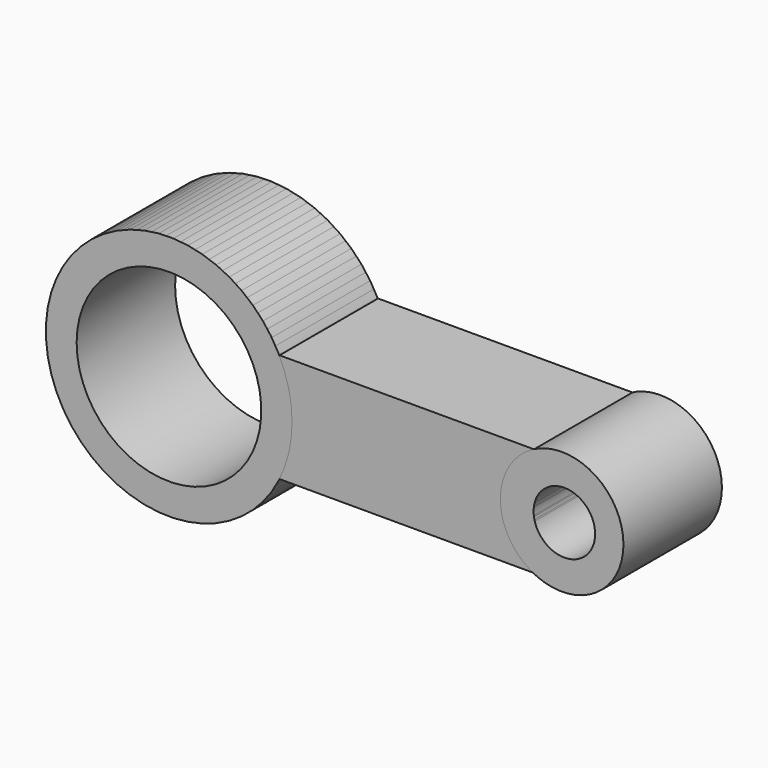
from build123d import *

# Parameters (mm, degrees)
F3_DEPTH   = 12.7
F0_R       = 12.7
F0_R_2     = 6.35
F5_D       = 19.05
F5_DEPTH   = 25.4
F5_TIP     = 5.7231973962
F5_2_D     = 19.05
F5_2_DEPTH = 25.4
F5_2_TIP   = 5.7231973962
F7_D       = 6.35
F7_DEPTH   = 12.7
F7_TIP     = 1.9077324654
F7_2_D     = 6.35
F7_2_DEPTH = 12.7
F7_2_TIP   = 1.9077324654


with BuildPart() as f3:
    # F1 (on face) → F3 (new body)
    with BuildSketch(Plane.XZ):
        with BuildLine():
            Line((37.7772264183, 5.648068618), (11.4167341962, 5.648068618))
            Line((11.4167341962, 5.648068618), (11.4167341962, 5.5631088694))
            ThreePointArc((11.4167341962, 5.5631088694), (12.3750257433, 2.8545994209), (12.7, 0))
            ThreePointArc((12.7, 0), (12.3750257433, -2.8545994209), (11.4167341962, -5.5631088694))
            Line((11.4167341962, -5.5631088694), (11.4167341962, -5.5927410722))
            Line((11.4167341962, -5.5927410722), (37.7772264183, -5.5927410722))
            Line((37.7772264183, -5.5927410722), (37.7772264183, 5.648068618))
        make_face()
        with BuildLine():
            ThreePointArc((12.7, 0), (12.3750257433, 2.8545994209), (11.4167341962, 5.5631088694))
            Line((11.4167341962, 5.5631088694), (11.4167341962, -5.5631088694))
            ThreePointArc((11.4167341962, -5.5631088694), (12.3750257433, -2.8545994209), (12.7, 0))
        make_face()
        with BuildLine():
            Line((11.4167341962, -5.5631088694), (11.4167341962, 5.5631088694))
            ThreePointArc((11.4167341962, 5.5631088694), (-12.7, 0), (11.4167341962, -5.5631088694))
        make_face()
    extrude(amount=F3_DEPTH)

    # F5
    with Locations(Plane(origin=(0, 0, 0), x_dir=(1, 0, 0), z_dir=(0, 1, 0))):
        with Locations((0, 0)):
            Hole(F5_D / 2, depth=F5_DEPTH)
            with Locations((0, 0, -(F5_DEPTH + F5_TIP / 2))):  # 118° drill point
                Cone(0, F5_D / 2, F5_TIP, mode=Mode.SUBTRACT)

    # F7
    with Locations(Plane(origin=(0, 0, 0), x_dir=(1, 0, 0), z_dir=(0, 1, 0))):
        with Locations((40.7965891063, 0)):
            Hole(F7_D / 2, depth=F7_DEPTH)
            with Locations((0, 0, -(F7_DEPTH + F7_TIP / 2))):  # 118° drill point
                Cone(0, F7_D / 2, F7_TIP, mode=Mode.SUBTRACT)


with BuildPart() as f3b:
    # F0 (on Front) → F3, piece 2 (new body)
    with BuildSketch(Plane.XZ):
        Circle(F0_R)
    extrude(amount=F3_DEPTH)

    # F5#2
    with Locations(Plane(origin=(0, 0, 0), x_dir=(1, 0, 0), z_dir=(0, 1, 0))):
        with Locations((0, 0)):
            Hole(F5_2_D / 2, depth=F5_2_DEPTH)
            with Locations((0, 0, -(F5_2_DEPTH + F5_2_TIP / 2))):  # 118° drill point
                Cone(0, F5_2_D / 2, F5_2_TIP, mode=Mode.SUBTRACT)


with BuildPart() as f3c:
    # F0 (on Front) → F3, piece 3 (new body)
    with BuildSketch(Plane.XZ):
        with Locations((40.5429568411, 0)):
            Circle(F0_R_2)
    extrude(amount=F3_DEPTH)

    # F7#2
    with Locations(Plane(origin=(0, 0, 0), x_dir=(1, 0, 0), z_dir=(0, 1, 0))):
        with Locations((40.7965891063, 0)):
            Hole(F7_2_D / 2, depth=F7_2_DEPTH)
            with Locations((0, 0, -(F7_2_DEPTH + F7_2_TIP / 2))):  # 118° drill point
                Cone(0, F7_2_D / 2, F7_2_TIP, mode=Mode.SUBTRACT)


solid = Compound([f3.part, f3b.part, f3c.part])
